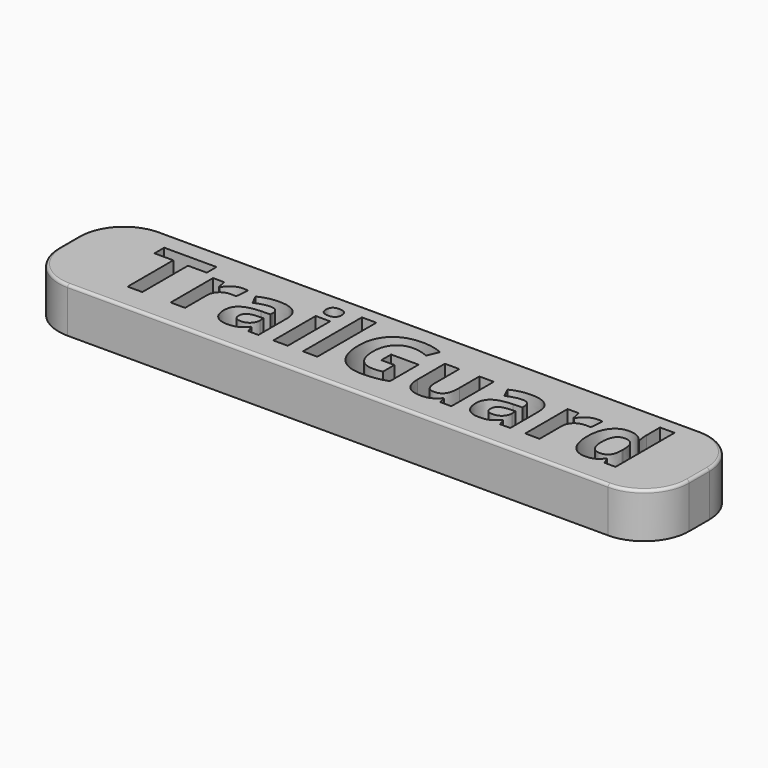
from build123d import *

# Parameters (mm, degrees)
F1_DEPTH     = 5
F2_TEXT_SIZE = 10.7728979654
F3_DEPTH     = 3
F4_R         = 0.3


# Not quite as in the source:
# - Text() gives the source's letters only with a copy of the font that has no kerning and outlines rounded to 1/6400 em; it was checked with that copy


with BuildPart() as f1:
    # F0 (on Top) → F1 (new body)
    with BuildSketch(Plane.XY):
        with BuildLine():
            ThreePointArc((35, 1.4), (33.5355339059, 4.9355339059), (30, 6.4))
            Line((30, 6.4), (-30, 6.4))
            ThreePointArc((-30, 6.4), (-33.5355339059, 4.9355339059), (-35, 1.4))
            Line((-35, 1.4), (-35, -1.4))
            ThreePointArc((-35, -1.4), (-33.5355339059, -4.9355339059), (-30, -6.4))
            Line((-30, -6.4), (30, -6.4))
            ThreePointArc((30, -6.4), (33.5355339059, -4.9355339059), (35, -1.4))
            Line((35, -1.4), (35, 1.4))
        make_face()
    extrude(amount=-F1_DEPTH)

    # F2 (on face) → F3 (cut)
    with BuildSketch(Plane.XY):
        with Locations((-28.0095338821, -3.4473263659)):
            Text('TrailGuard', F2_TEXT_SIZE, font='Open Sans', font_style=FontStyle.BOLD, text_align=(TextAlign.LEFT, TextAlign.BOTTOM))
    extrude(amount=-F3_DEPTH, mode=Mode.SUBTRACT)

    # F4
    f4_edges = [f1.edges().sort_by_distance(p)[0] for p in [
        (0, 6.4, 0),
        (0, -6.4, 0),
        (33.535534, -4.935534, 0),
        (35, 0, 0),
        (33.535534, 4.935534, 0),
        (-33.535534, 4.935534, 0),
        (-35, 0, 0),
        (-33.535534, -4.935534, 0),
    ]]
    fillet(f4_edges, radius=F4_R)


solid = f1.part
